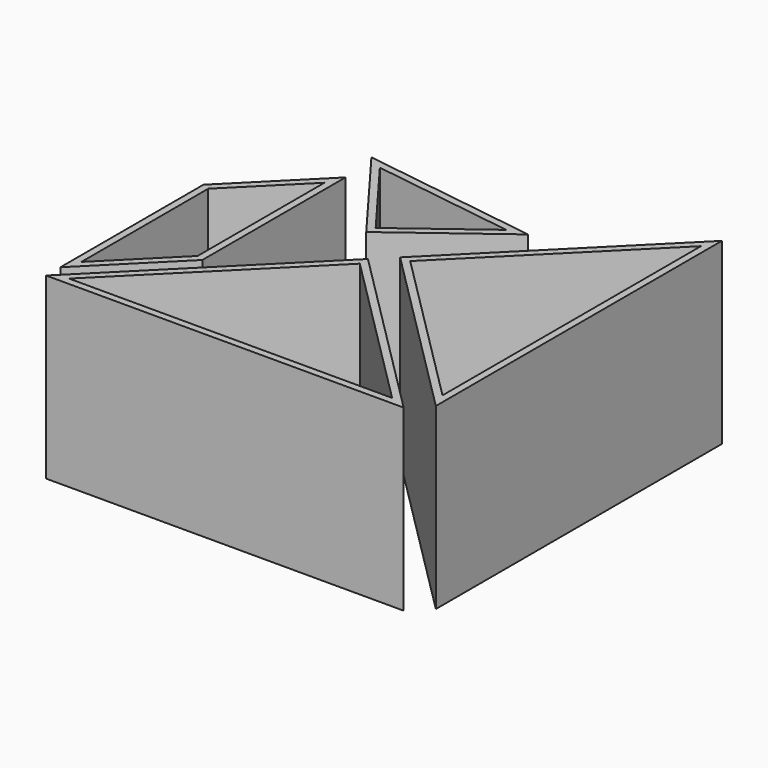
from build123d import *

# Parameters (mm, degrees)
F1_DEPTH = 50
F2_T     = -2
F2_2_T   = -2
F2_3_T   = -2
F2_4_T   = -2


# Not quite as in the source:
# - a feature names something its author has since deleted; it is built from what else it names


with BuildPart() as f1:
    # F0 (on Top) → F1 (new body)
    with BuildSketch(Plane.XY):
        Polygon((-16.5389066256, -1.8107631532), (-66.5389066256, -51.8107631532), (-16.5389066256, -101.8107631532), align=None)
    extrude(amount=F1_DEPTH)

    # F2
    f2_openings = [f1.faces().sort_by_distance(p)[0] for p in [
        (-33.205573, -51.810763, 50),
    ]]
    offset(amount=F2_T, openings=f2_openings)


with BuildPart() as f1b:
    # F0 (on Top) → F1, piece 2 (new body)
    with BuildSketch(Plane.XY):
        Polygon((-100.9843560544, -18.7777006427), (-79.7953103328, -47.0800740662), (-51.4929369092, -25.8910283446), align=None)
    extrude(amount=F1_DEPTH)

    # F2#3
    f2_3_openings = [f1b.faces().sort_by_distance(p)[0] for p in [
        (-77.424201, -30.582934, 50),
    ]]
    offset(amount=F2_3_T, openings=f2_3_openings)


with BuildPart() as f1c:
    # F0 (on Top) → F1, piece 3 (new body)
    with BuildSketch(Plane.XY):
        Polygon((-99.47348535, -29.7453418775), (-121.5389066256, -51.8107631532), (-121.5389066256, -101.8107631532), (-99.47348535, -79.7453418775), align=None)
    extrude(amount=F1_DEPTH)

    # F2#4
    f2_4_openings = [f1c.faces().sort_by_distance(p)[0] for p in [
        (-110.506196, -65.778053, 50),
    ]]
    offset(amount=F2_4_T, openings=f2_4_openings)


with BuildPart() as f1d:
    # F0 (on Top) → F1, piece 4 (new body)
    with BuildSketch(Plane.XY):
        Polygon((-71.5389066256, -56.8107631532), (-121.5389066256, -106.8107631532), (-21.5389066256, -106.8107631532), align=None)
    extrude(amount=F1_DEPTH)

    # F2#2
    f2_2_openings = [f1d.faces().sort_by_distance(p)[0] for p in [
        (-71.538907, -90.144096, 50),
    ]]
    offset(amount=F2_2_T, openings=f2_2_openings)


solid = Compound([f1.part, f1b.part, f1c.part, f1d.part])
